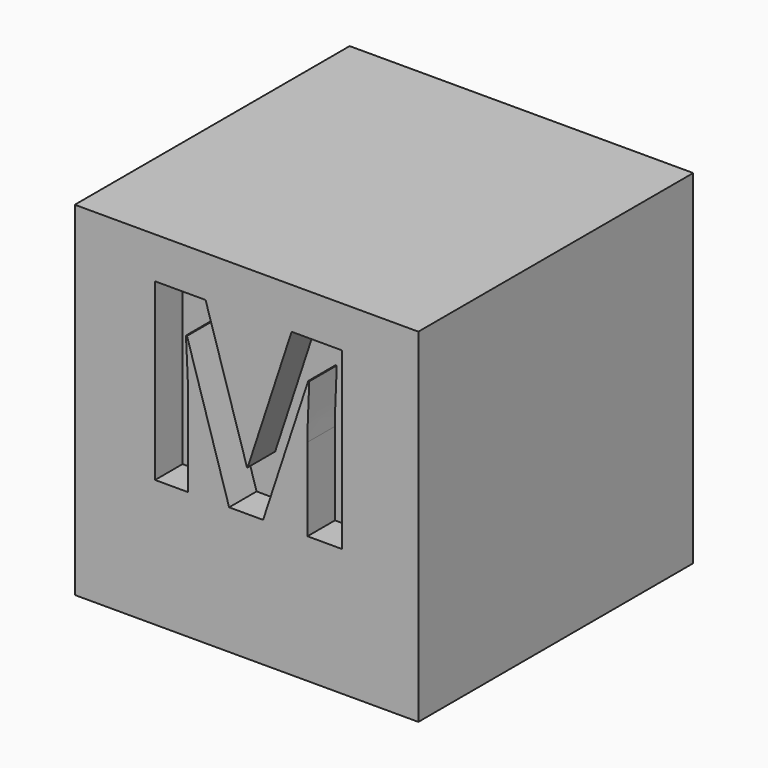
from build123d import *

# Parameters (mm, degrees)
F0_W         = 10
F0_H         = 10
F1_DEPTH     = 10
F2_TEXT_SIZE = 7.1303847815
F3_DEPTH     = 1


# Not quite as in the source:
# - Text() gives the source's letters only with a copy of the font that has no kerning and outlines rounded to 1/6400 em; it was checked with that copy


with BuildPart() as f1:
    # F0 (on Top) → F1 (new body)
    with BuildSketch(Plane.XY):
        Rectangle(F0_W, F0_H)
    extrude(amount=F1_DEPTH)

    # F2 (on face) → F3 (cut)
    with BuildSketch(Plane.XZ.offset(5)):
        with Locations((-3.3034915105, 3.7075350992)):
            Text('M', F2_TEXT_SIZE, font='Open Sans', font_style=FontStyle.BOLD, text_align=(TextAlign.LEFT, TextAlign.BOTTOM))
    extrude(amount=-F3_DEPTH, mode=Mode.SUBTRACT)


solid = f1.part
